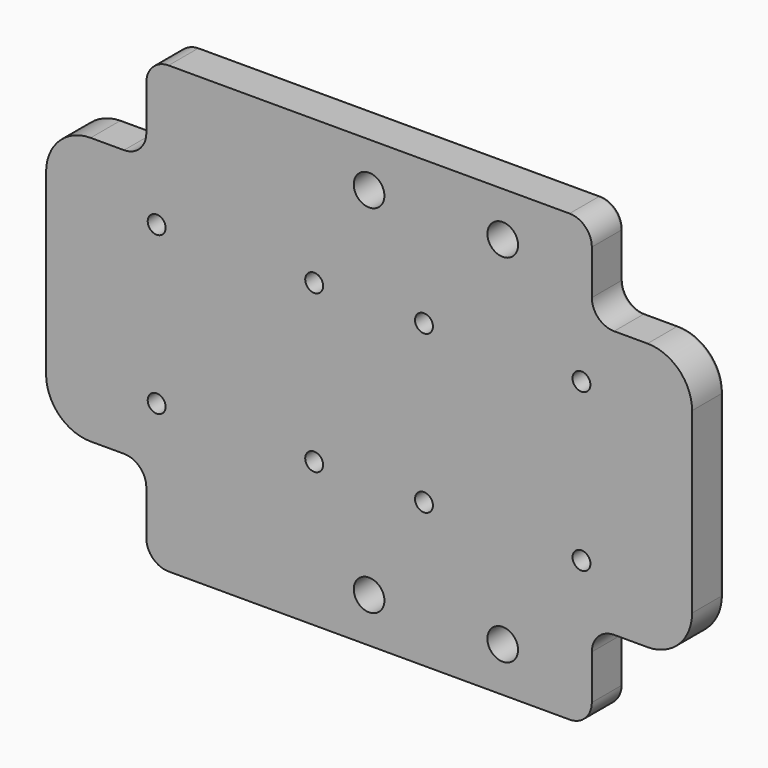
from build123d import *

# Parameters (mm, degrees)
F0_W     = 184.15
F0_H     = 76.2
F1_DEPTH = 11.176
F2_R     = 12.7
F3_W     = 127
F3_H     = 25.4
F4_DEPTH = 11.176
F5_R     = 6.35
F7_D     = 5.1054
F8_R     = 0.8255
F10_D    = 8.7376


# Not quite as in the source:
# - a feature names something its author has since deleted; it is built from what else it names


with BuildPart() as f1:
    # F0 (on Front) → F1 (new body)
    with BuildSketch(Plane.XZ):
        Rectangle(F0_W, F0_H)
    extrude(amount=F1_DEPTH)

    # F2
    f2_edges = [f1.edges().sort_by_distance(p)[0] for p in [
        (92.075, -5.588, 38.1),
        (92.075, -5.588, -38.1),
        (-92.075, -5.588, -38.1),
        (-92.075, -5.588, 38.1),
    ]]
    fillet(f2_edges, radius=F2_R)

    # F3 (on Front) → F4 (join)
    with BuildSketch(Plane.XZ):
        with Locations((0, 50.8)):
            Rectangle(F3_W, F3_H)
        with Locations((0, -50.8)):
            Rectangle(F3_W, F3_H)
    extrude(amount=F4_DEPTH)

    # F5
    f5_edges = [f1.edges().sort_by_distance(p)[0] for p in [
        (-63.5, -5.588, 63.5),
        (-63.5, -5.588, 38.1),
        (63.5, -5.588, 63.5),
        (63.5, -5.588, 38.1),
        (-63.5, -5.588, -63.5),
        (63.5, -5.588, -63.5),
        (63.5, -5.588, -38.1),
        (-63.5, -5.588, -38.1),
    ]]
    fillet(f5_edges, radius=F5_R)

    # F7 (through all)
    with Locations(Plane(origin=(0, 0, 0), x_dir=(-1, 0, 0), z_dir=(0, 1, 0))):
        with Locations((-60.5506403027, 22.4506403027), (-15.6493596973, 22.4506403027), (-60.5506403027, -22.4506403027), (-15.6493596973, -22.4506403027), (15.6493596973, 22.4506403027), (15.6493596973, -22.4506403027), (60.5506403027, 22.4506403027), (60.5506403027, -22.4506403027)):
            Hole(F7_D / 2)

    # F8
    f8_edges = [f1.edges().sort_by_distance(p)[0] for p in [
        (0, 0, 63.5),
    ]]
    fillet(f8_edges, radius=F8_R)

    # F10 (through all)
    with Locations(Plane(origin=(0, 0, 0), x_dir=(-1, 0, 0), z_dir=(0, 1, 0))):
        with Locations((-38.1, 50.8), (0, 50.8), (-38.1, -50.8), (0, -50.8)):
            Hole(F10_D / 2)


solid = f1.part
